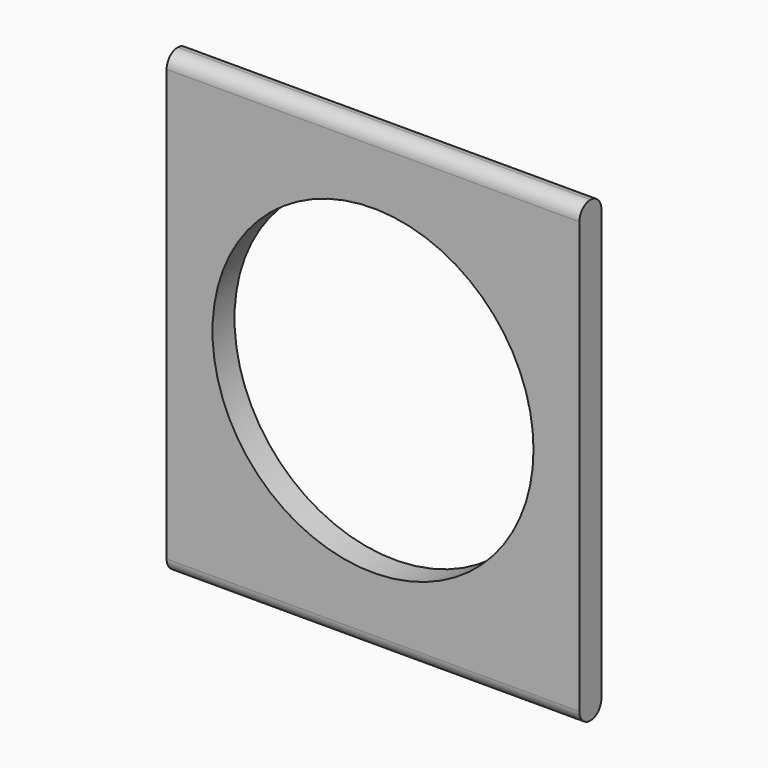
from build123d import *

# Parameters (mm, degrees)
F1_DEPTH     = 22.5
F2_R         = 18.6
F3_DEPTH     = 6
F4_R         = 17.5
F5_DEPTH     = 3
F7_DEPTH     = 3
F8_DEPTH     = 3
F14_DEPTH    = 3
F9_T1_DEPTH  = 3
F9_T6_DEPTH  = 3
F9_T11_DEPTH = 3
F15_W        = 6
F15_H        = 97.4
F10_DEPTH    = 45.001
F11_R        = 1.49999


# Not quite as in the source:
# - a fillet or chamfer that OpenCascade refuses, or shapes differently, is made with other operations: its cross-section is extruded or revolved along the edge and cut away or added
# - a fillet or chamfer is up to 0.001 mm smaller than in the source, because OpenCascade refuses the exact size


with BuildPart() as f1:
    # F0 (on Right) → F1 (new body, symmetric)
    with BuildSketch(Plane.YZ):
        Polygon((0, -25), (0, 25), (-3, 25), (-3, 21.25), (-9, 21.25), (-9, -21.25), (-3, -21.25), (-3, -25), align=None)
    extrude(amount=F1_DEPTH, both=True)

    # F2 (on face) → F3 (cut)
    with BuildSketch(Plane.XZ.offset(9)):
        Circle(F2_R)
    extrude(amount=-F3_DEPTH, mode=Mode.SUBTRACT)

    # F4 (on face) → F5 (cut, through all)
    with BuildSketch(Plane.XZ.offset(3)):
        Circle(F4_R)
    extrude(amount=-F5_DEPTH, mode=Mode.SUBTRACT)

    # F6 (on face) → F7 (join)
    with BuildSketch(Plane.XZ.offset(9)):
        with BuildLine():
            Line((-1.6773361726, 21.1145450883), (-1.5, 21.05))
            Line((-1.5, 21.05), (2.8857066002, 21.05))
            Line((2.8857066002, 21.05), (-1.1643059576, 22.5240840195))
            ThreePointArc((-1.1643059576, 22.5240840195), (-1.8221335094, 23.4812290467), (-1.1313028087, 24.4148331565))
            Line((-1.1313028087, 24.4148331565), (1.1823725422, 25.1665918487))
            ThreePointArc((1.1823725422, 25.1665918487), (2.9098300563, 27.5442331395), (1.1823725422, 29.9218744302))
            Line((1.1823725422, 29.9218744302), (-2.6423503277, 31.1646022233))
            ThreePointArc((-2.6423503277, 31.1646022233), (-3.3282367753, 32.0148264964), (-2.8268835217, 32.9853760566))
            Line((-2.8268835217, 32.9853760566), (3.5672088043, 36.6139176646))
            ThreePointArc((3.5672088043, 36.6139176646), (4.8205919381, 39.0402915651), (3.1058758193, 41.165852248))
            Line((3.1058758193, 41.165852248), (-0.0769036922, 42.2))
            Line((-0.0769036922, 42.2), (-4.9310056584, 42.2))
            Line((-4.9310056584, 42.2), (2.6423503277, 39.7392674735))
            ThreePointArc((2.6423503277, 39.7392674735), (3.3282367753, 38.8890432004), (2.8268835217, 37.9184936402))
            Line((2.8268835217, 37.9184936402), (-3.5672088043, 34.2899520321))
            ThreePointArc((-3.5672088043, 34.2899520321), (-4.8205919381, 31.8635781317), (-3.1058758193, 29.7380174488))
            Line((-3.1058758193, 29.7380174488), (0.7188470506, 28.4952896558))
            ThreePointArc((0.7188470506, 28.4952896558), (1.4098300563, 27.5442331395), (0.7188470506, 26.5931766232))
            Line((0.7188470506, 26.5931766232), (-1.5948283002, 25.841417931))
            ThreePointArc((-1.5948283002, 25.841417931), (-3.3219050522, 23.5074076563), (-1.6773361726, 21.1145450883))
        make_face()
        with BuildLine():
            Line((3.5672088043, -36.6139176646), (-2.8268835217, -32.9853760566))
            ThreePointArc((-2.8268835217, -32.9853760566), (-3.3282367753, -32.0148264964), (-2.6423503277, -31.1646022233))
            Line((-2.6423503277, -31.1646022233), (1.1823725422, -29.9218744302))
            ThreePointArc((1.1823725422, -29.9218744302), (2.9098300563, -27.5442331395), (1.1823725422, -25.1665918487))
            Line((1.1823725422, -25.1665918487), (-1.1313028087, -24.4148331565))
            ThreePointArc((-1.1313028087, -24.4148331565), (-1.8221335094, -23.4812290467), (-1.1643059576, -22.5240840195))
            Line((-1.1643059576, -22.5240840195), (2.8857066002, -21.05))
            Line((2.8857066002, -21.05), (-1.5, -21.05))
            Line((-1.5, -21.05), (-1.6773361726, -21.1145450883))
            ThreePointArc((-1.6773361726, -21.1145450883), (-3.3219050522, -23.5074076563), (-1.5948283002, -25.841417931))
            Line((-1.5948283002, -25.841417931), (0.7188470506, -26.5931766232))
            ThreePointArc((0.7188470506, -26.5931766232), (1.4098300563, -27.5442331395), (0.7188470506, -28.4952896558))
            Line((0.7188470506, -28.4952896558), (-3.1058758193, -29.7380174488))
            ThreePointArc((-3.1058758193, -29.7380174488), (-4.8205919381, -31.8635781317), (-3.5672088043, -34.2899520321))
            Line((-3.5672088043, -34.2899520321), (2.8268835217, -37.9184936402))
            ThreePointArc((2.8268835217, -37.9184936402), (3.3282367753, -38.8890432004), (2.6423503277, -39.7392674735))
            Line((2.6423503277, -39.7392674735), (-4.9310056584, -42.2))
            Line((-4.9310056584, -42.2), (-0.0769036922, -42.2))
            Line((-0.0769036922, -42.2), (3.1058758193, -41.165852248))
            ThreePointArc((3.1058758193, -41.165852248), (4.8205919381, -39.0402915651), (3.5672088043, -36.6139176646))
        make_face()
    extrude(amount=-F7_DEPTH)

    # F12 (on face) → F8 (join)
    with BuildSketch(Plane.XZ.offset(9)):
        with BuildLine():
            Line((-10.0039546753, 45.1082380117), (-10.0039546753, 41.7))
            Line((-10.0039546753, 41.7), (-2.5039546753, 41.7))
            Line((-2.5039546753, 41.7), (4.9960453247, 41.7))
            Line((4.9960453247, 41.7), (4.9960453247, 45.1082380117))
            ThreePointArc((4.9960453247, 45.1082380117), (4.9619908828, 45.2896070742), (4.8644663773, 45.446270448))
            ThreePointArc((4.8644663773, 45.446270448), (-2.5039546753, 48.6856217223), (-9.872375728, 45.446270448))
            ThreePointArc((-9.872375728, 45.446270448), (-9.9699002335, 45.2896070742), (-10.0039546753, 45.1082380117))
        make_face()
        with BuildLine():
            Line((4.9960453247, -41.7), (-10.0039546753, -41.7))
            Line((-10.0039546753, -41.7), (-10.0039546753, -45.1082380117))
            ThreePointArc((-10.0039546753, -45.1082380117), (-9.9699002335, -45.2896070742), (-9.872375728, -45.446270448))
            ThreePointArc((-9.872375728, -45.446270448), (-2.5039546753, -48.6856217223), (4.8644663773, -45.446270448))
            ThreePointArc((4.8644663773, -45.446270448), (4.9619908828, -45.2896070742), (4.9960453247, -45.1082380117))
            Line((4.9960453247, -45.1082380117), (4.9960453247, -41.7))
        make_face()
    extrude(amount=-F8_DEPTH)

    # F13 (on face) → F14 (join)
    with BuildSketch(Plane(origin=(0, -6, 0), x_dir=(-1, 0, 0), z_dir=(0, 1, 0))):
        Polygon((-4.9960453247, 41.7), (10.0039546753, 41.7), (10.0039546753, 41.9), (9.0039546753, 42.9), (8.0039546753, 41.9), (7.0039546753, 42.9), (6.0039546753, 41.9), (5.0039546753, 42.9), (4.0039546753, 41.9), (3.0039546753, 42.9), (2.0039546753, 41.9), (1.0039546753, 42.9), (0.0039546753, 41.9), (-0.9960453247, 42.9), (-1.9960453247, 41.9), (-2.9960453247, 42.9), (-3.9960453247, 41.9), (-4.9960453247, 42.9), align=None)
        Polygon((-4.9960453247, -41.7), (-4.9960453247, -42.9), (-3.9960453247, -41.9), (-2.9960453247, -42.9), (-1.9960453247, -41.9), (-0.9960453247, -42.9), (0.0039546753, -41.9), (1.0039546753, -42.9), (2.0039546753, -41.9), (3.0039546753, -42.9), (4.0039546753, -41.9), (5.0039546753, -42.9), (6.0039546753, -41.9), (7.0039546753, -42.9), (8.0039546753, -41.9), (9.0039546753, -42.9), (10.0039546753, -41.9), (10.0039546753, -41.7), align=None)
    extrude(amount=F14_DEPTH)

    # F9: fillet of radius 1 on 8 edges, made by hand

    # F9_s2 → F9_t1 (join)
    with BuildSketch(Plane.XZ.offset(6)):
        with BuildLine():
            ThreePointArc((-3.1671397399, 22.5967933258), (-3.2844738139, 21.6785077979), (-4.1050813101, 21.25))
            Line((-4.1050813101, 21.25), (-1.9838334832, 21.25))
            ThreePointArc((-1.9838334832, 21.25), (-2.7003635819, 21.813678492), (-3.1671397399, 22.5967933258))
        make_face()
        with BuildLine():
            ThreePointArc((2.1705179537, 21.3103073792), (2.3388899194, 21.265192247), (2.5125380971, 21.25))
            Line((2.5125380971, 21.25), (2.3362111164, 21.25))
            Line((2.3362111164, 21.25), (2.1705179537, 21.3103073792))
        make_face()
        with BuildLine():
            ThreePointArc((-3.2415313358, 41.6510565163), (-3.3941138651, 41.6876883406), (-3.5505483302, 41.7))
            Line((-3.5505483302, 41.7), (-3.3921638899, 41.7))
            Line((-3.3921638899, 41.7), (-3.2415313358, 41.6510565163))
        make_face()
        with BuildLine():
            ThreePointArc((-3.1671397399, -22.5967933258), (-3.2844738139, -21.6785077979), (-4.1050813101, -21.25))
            Line((-4.1050813101, -21.25), (-1.9838334832, -21.25))
            ThreePointArc((-1.9838334832, -21.25), (-2.7003635819, -21.813678492), (-3.1671397399, -22.5967933258))
        make_face()
        with BuildLine():
            ThreePointArc((-3.5505483302, -41.7), (-3.3941138651, -41.6876883406), (-3.2415313358, -41.6510565163))
            Line((-3.2415313358, -41.6510565163), (-3.3921638899, -41.7))
            Line((-3.3921638899, -41.7), (-3.5505483302, -41.7))
        make_face()
        with BuildLine():
            ThreePointArc((2.1705179537, -21.3103073792), (2.3388899194, -21.265192247), (2.5125380971, -21.25))
            Line((2.5125380971, -21.25), (2.3362111164, -21.25))
            Line((2.3362111164, -21.25), (2.1705179537, -21.3103073792))
        make_face()
    extrude(amount=F9_T1_DEPTH)


with BuildPart() as f9_tool4:
    # F9_s5 → F9_t6 (new body)
    with BuildSketch(Plane.XZ.offset(9)):
        with BuildLine():
            ThreePointArc((5.265067062, 41.7), (4.3857987751, 41.1763268621), (4.4274288538, 40.1537745592))
            Line((4.4274288538, 40.1537745592), (4.343665033, 40.0991520151))
            ThreePointArc((4.343665033, 40.0991520151), (3.0749741198, 41.0707465963), (1.431036377, 41.6048943484))
            Line((1.431036377, 41.6048943484), (1.4619380764, 41.8))
            Line((1.4619380764, 41.8), (5.265067062, 41.8))
            Line((5.265067062, 41.8), (5.265067062, 41.7))
        make_face()
    extrude(amount=-F9_T6_DEPTH)

    split(bisect_by=Plane.YZ.offset(4.9960453247), keep=Keep.BOTTOM)


with BuildPart() as f1_1:
    add(f1.part)

    # F9_t3: union F9_tool4
    add(f9_tool4.part)


with BuildPart() as f9_tool9:
    # F9_s10 → F9_t11 (new body)
    with BuildSketch(Plane.XZ.offset(6)):
        with BuildLine():
            ThreePointArc((4.4274288538, -40.1537745592), (4.3857987751, -41.1763268621), (5.265067062, -41.7))
            Line((5.265067062, -41.7), (5.265067062, -41.8))
            Line((5.265067062, -41.8), (1.4619380764, -41.8))
            Line((1.4619380764, -41.8), (1.431036377, -41.6048943484))
            ThreePointArc((1.431036377, -41.6048943484), (3.0749741198, -41.0707465963), (4.343665033, -40.0991520151))
            Line((4.343665033, -40.0991520151), (4.4274288538, -40.1537745592))
        make_face()
    extrude(amount=F9_T11_DEPTH)

    split(bisect_by=Plane.YZ.offset(4.9960453247), keep=Keep.BOTTOM)


with BuildPart() as f1_2:
    add(f1_1.part)

    # F9_t8: union F9_tool9
    add(f9_tool9.part)

    # F15 (on face) → F10 (cut, through all)
    with BuildSketch(Plane.YZ.offset(22.5)):
        with Locations((-6, 0)):
            Rectangle(F15_W, F15_H)
    extrude(amount=-F10_DEPTH, mode=Mode.SUBTRACT)

    # F11 (radius 1.5 in the source; OpenCascade refuses exactly that, so slightly less here)
    f11_edges = [f1_2.edges().sort_by_distance(p)[0] for p in [
        (0, -3, 25),
        (0, 0, 25),
        (0, -3, -25),
        (0, 0, -25),
    ]]
    fillet(f11_edges, radius=F11_R)


solid = f1_2.part
